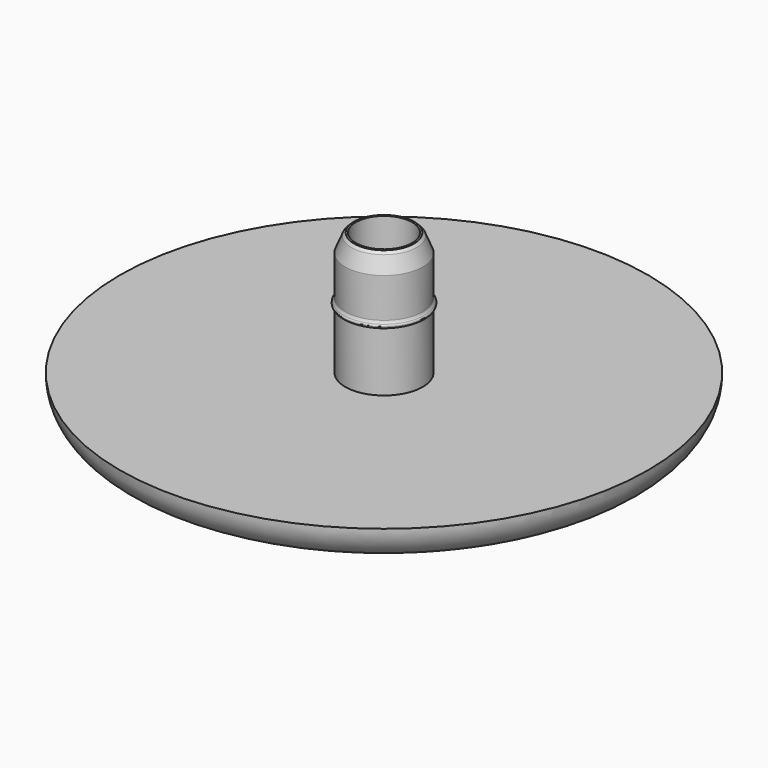
from build123d import *

# Parameters (mm, degrees)
F0_R     = 2.2
F1_DEPTH = 7
F2_T     = -0.6
F0_R_2   = 15
F3_DEPTH = 2
F4_R     = 1.99999
F7_SIZE  = 0.5
F8_SIZE  = 0.5
F9_R     = 0.2


# Not quite as in the source:
# - a fillet or chamfer is up to 0.001 mm smaller than in the source, because OpenCascade refuses the exact size


with BuildPart() as f1:
    # F0 (on Top) → F1 (new body)
    with BuildSketch(Plane.XY):
        Circle(F0_R)
    extrude(amount=F1_DEPTH)

    # F2
    f2_openings = [f1.faces().sort_by_distance(p)[0] for p in [
        (0, 0, 7),
    ]]
    offset(amount=F2_T, openings=f2_openings)

    # F0 (on Top) → F3 (join)
    with BuildSketch(Plane.XY):
        Circle(F0_R_2)
        Circle(F0_R, mode=Mode.SUBTRACT)
        Circle(F0_R)
    extrude(amount=-F3_DEPTH)

    # F4 (radius 2 in the source; OpenCascade refuses exactly that, so slightly less here)
    f4_edges = [f1.edges().sort_by_distance(p)[0] for p in [
        (-15, 0, -2),
    ]]
    fillet(f4_edges, radius=F4_R)

    # F5 (on Front) → F6 (revolve)
    with BuildSketch(Plane.XZ):
        with BuildLine():
            ThreePointArc((2.075, 3.5), (2.1116116524, 3.4116116524), (2.2, 3.375))
            Line((2.2, 3.375), (2.2, 3.5))
            Line((2.2, 3.5), (2.075, 3.5))
        make_face()
        with BuildLine():
            Line((2.2, 3.5), (2.2, 3.375))
            ThreePointArc((2.2, 3.375), (2.2883883476, 3.4116116524), (2.325, 3.5))
            ThreePointArc((2.325, 3.5), (2.2, 3.625), (2.075, 3.5))
            Line((2.075, 3.5), (2.2, 3.5))
        make_face()
    revolve(axis=Axis((0, 0, 1.75), (0, 0, 1)))

    # F7
    f7_edges = [f1.edges().sort_by_distance(p)[0] for p in [
        (-2.2, 0, 7),
    ]]
    chamfer(f7_edges, length=F7_SIZE)

    # F8
    f8_edges = [f1.edges().sort_by_distance(p)[0] for p in [
        (-2.2, 0, 6.5),
    ]]
    chamfer(f8_edges, length=F8_SIZE)

    # F9
    f9_edges = [f1.edges().sort_by_distance(p)[0] for p in [
        (-2.2, 0, 3.625),
    ]]
    fillet(f9_edges, radius=F9_R)


solid = f1.part
